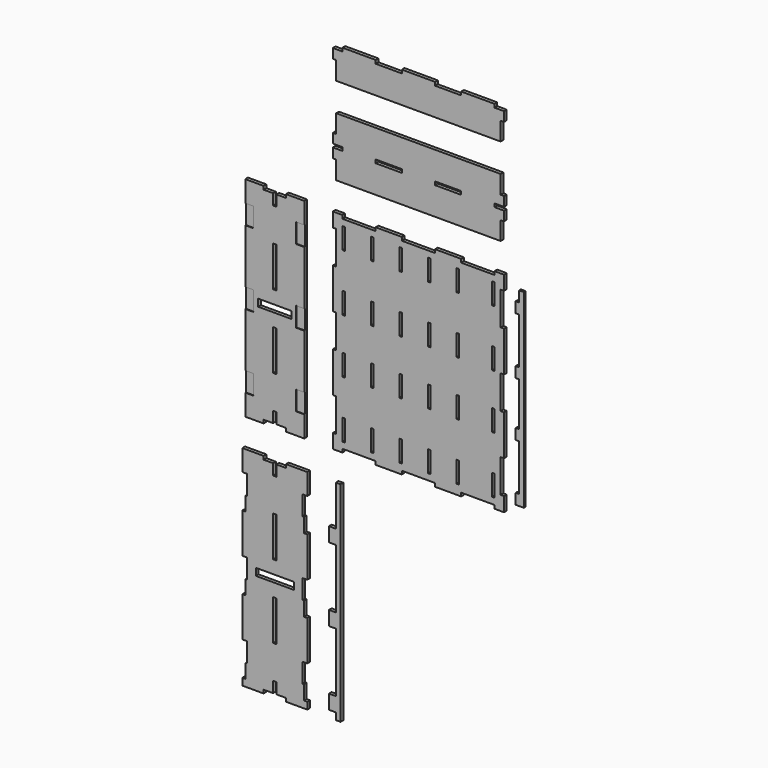
from build123d import *

# Parameters (mm, degrees)
F1_W     = 139.7
F1_H     = 18.034
F1_W_2   = 18.034
F1_H_2   = 50.8
F2_DEPTH = 18.034
F1_W_3   = 12.192
F1_H_3   = 113.5253
F1_H_4   = 215.9
F1_W_4   = 203.2
F1_H_5   = 38.1
F1_W_5   = 37.084
F1_H_6   = 76.2
F1_W_6   = 25.4
F1_H_7   = 217.17
F1_H_8   = 36.83
F1_W_7   = 177.8
F1_H_9   = 56.76265
F3_DEPTH = 12.192
F1_W_8   = 43.7134
F1_H_10  = 104.14
F4_DEPTH = 14.7574


# Not quite as in the source:
# - a variable given as a bare number and used for a length is read in inches; the dataset says mm whatever the document's units were
# - a feature names something its author has since deleted; it is built from what else it names


with BuildPart() as f2:
    # F1 (on Front) → F2 (new body)
    with BuildSketch(Plane.XZ):
        Polygon((439.166, 1026.668), (-439.166, 1026.668), (-439.166, 928.751), (-439.166, 877.951), (-406.4, 877.951), (-406.4, 859.917), (-439.166, 859.917), (-439.166, 809.117), (-439.166, 711.2), (439.166, 711.2), (439.166, 809.117), (439.166, 859.917), (406.4, 859.917), (406.4, 877.951), (439.166, 877.951), (439.166, 928.751), align=None)
        with Locations((-158.75, 868.934)):
            Rectangle(F1_W, F1_H, mode=Mode.SUBTRACT)
        with Locations((158.75, 868.934)):
            Rectangle(F1_W, F1_H, mode=Mode.SUBTRACT)
        with Locations((-448.183, 903.351)):
            Rectangle(F1_W_2, F1_H_2)
        with Locations((-448.183, 834.517)):
            Rectangle(F1_W_2, F1_H_2)
        with Locations((448.183, 903.351)):
            Rectangle(F1_W_2, F1_H_2)
        with Locations((448.183, 834.517)):
            Rectangle(F1_W_2, F1_H_2)
    extrude(amount=F2_DEPTH)


with BuildPart() as f2b:
    # F1 (on Front) → F2, piece 2 (new body)
    with BuildSketch(Plane.XZ):
        Polygon((-406.4, 558.8), (-457.2, 558.8), (-457.2, 482.6), (-439.166, 482.6), (-439.166, 304.8), (-457.2, 304.8), (-457.2, 88.9), (-439.166, 88.9), (-439.166, -88.9), (-457.2, -88.9), (-457.2, -304.8), (-439.166, -304.8), (-439.166, -482.6), (-457.2, -482.6), (-457.2, -558.8), (-406.4, -558.8), (-406.4, -540.766), (-228.6, -540.766), (-228.6, -558.8), (-88.9, -558.8), (-88.9, -540.766), (88.9, -540.766), (88.9, -558.8), (228.6, -558.8), (228.6, -540.766), (406.4, -540.766), (406.4, -558.8), (457.2, -558.8), (457.2, -482.6), (439.166, -482.6), (439.166, -304.8), (457.2, -304.8), (457.2, -88.9), (439.166, -88.9), (439.166, 88.9), (457.2, 88.9), (457.2, 304.8), (439.166, 304.8), (439.166, 482.6), (457.2, 482.6), (457.2, 558.8), (406.4, 558.8), (406.4, 540.766), (228.6, 540.766), (228.6, 558.8), (88.9, 558.8), (88.9, 540.766), (-88.9, 540.766), (-88.9, 558.8), (-228.6, 558.8), (-228.6, 540.766), (-406.4, 540.766), align=None)
        with Locations((-399.5293, -450.46265)):
            Rectangle(F1_W_3, F1_H_3, mode=Mode.SUBTRACT)
        with Locations((-247.1293, -450.46265)):
            Rectangle(F1_W_3, F1_H_3, mode=Mode.SUBTRACT)
        with Locations((-94.7293, -450.46265)):
            Rectangle(F1_W_3, F1_H_3, mode=Mode.SUBTRACT)
        with Locations((57.6707, -450.46265)):
            Rectangle(F1_W_3, F1_H_3, mode=Mode.SUBTRACT)
        with Locations((210.0707, -450.46265)):
            Rectangle(F1_W_3, F1_H_3, mode=Mode.SUBTRACT)
        with Locations((399.5293, -450.46265)):
            Rectangle(F1_W_3, F1_H_3, mode=Mode.SUBTRACT)
        with Locations((-399.5293, -145.66265)):
            Rectangle(F1_W_3, F1_H_3, mode=Mode.SUBTRACT)
        with Locations((-399.5293, 145.66265)):
            Rectangle(F1_W_3, F1_H_3, mode=Mode.SUBTRACT)
        with Locations((-247.1293, -145.66265)):
            Rectangle(F1_W_3, F1_H_3, mode=Mode.SUBTRACT)
        with Locations((-247.1293, 145.66265)):
            Rectangle(F1_W_3, F1_H_3, mode=Mode.SUBTRACT)
        with Locations((-399.5293, 450.46265)):
            Rectangle(F1_W_3, F1_H_3, mode=Mode.SUBTRACT)
        with Locations((-247.1293, 450.46265)):
            Rectangle(F1_W_3, F1_H_3, mode=Mode.SUBTRACT)
        with Locations((-94.7293, -145.66265)):
            Rectangle(F1_W_3, F1_H_3, mode=Mode.SUBTRACT)
        with Locations((-94.7293, 145.66265)):
            Rectangle(F1_W_3, F1_H_3, mode=Mode.SUBTRACT)
        with Locations((57.6707, -145.66265)):
            Rectangle(F1_W_3, F1_H_3, mode=Mode.SUBTRACT)
        with Locations((57.6707, 145.66265)):
            Rectangle(F1_W_3, F1_H_3, mode=Mode.SUBTRACT)
        with Locations((-94.7293, 450.46265)):
            Rectangle(F1_W_3, F1_H_3, mode=Mode.SUBTRACT)
        with Locations((57.6707, 450.46265)):
            Rectangle(F1_W_3, F1_H_3, mode=Mode.SUBTRACT)
        with Locations((210.0707, -145.66265)):
            Rectangle(F1_W_3, F1_H_3, mode=Mode.SUBTRACT)
        with Locations((210.0707, 145.66265)):
            Rectangle(F1_W_3, F1_H_3, mode=Mode.SUBTRACT)
        with Locations((399.5293, -145.66265)):
            Rectangle(F1_W_3, F1_H_3, mode=Mode.SUBTRACT)
        with Locations((399.5293, 145.66265)):
            Rectangle(F1_W_3, F1_H_3, mode=Mode.SUBTRACT)
        with Locations((210.0707, 450.46265)):
            Rectangle(F1_W_3, F1_H_3, mode=Mode.SUBTRACT)
        with Locations((399.5293, 450.46265)):
            Rectangle(F1_W_3, F1_H_3, mode=Mode.SUBTRACT)
    extrude(amount=F2_DEPTH)


with BuildPart() as f2c:
    # F1 (on Front) → F2, piece 3 (new body)
    with BuildSketch(Plane.XZ):
        Polygon((-439.166, 1276.985), (-439.166, 1179.068), (439.166, 1179.068), (439.166, 1276.985), (439.166, 1327.785), (406.4, 1327.785), (406.4, 1345.819), (228.6, 1345.819), (228.6, 1327.785), (88.9, 1327.785), (88.9, 1345.819), (-88.9, 1345.819), (-88.9, 1327.785), (-228.6, 1327.785), (-228.6, 1345.819), (-406.4, 1345.819), (-406.4, 1327.785), (-439.166, 1327.785), align=None)
        with Locations((448.183, 1302.385)):
            Rectangle(F1_W_2, F1_H_2)
        with Locations((-448.183, 1302.385)):
            Rectangle(F1_W_2, F1_H_2)
    extrude(amount=F2_DEPTH)


with BuildPart() as f2d:
    # F1 (on Front) → F2, piece 4 (new body)
    with BuildSketch(Plane.XZ):
        Polygon((-827.151, -711.2), (-940.943, -711.2), (-940.943, -824.23), (-915.543, -824.23), (-915.543, -928.37), (-922.909, -928.37), (-922.909, -1004.57), (-940.943, -1004.57), (-940.943, -1217.93), (-915.543, -1217.93), (-915.543, -1322.07), (-922.909, -1322.07), (-922.909, -1398.27), (-940.943, -1398.27), (-940.943, -1611.63), (-915.543, -1611.63), (-915.543, -1715.77), (-922.909, -1715.77), (-922.909, -1791.97), (-940.943, -1791.97), (-940.943, -1828.8), (-827.151, -1828.8), (-827.151, -1810.766), (-776.351, -1810.766), (-776.351, -1752.6), (-758.317, -1752.6), (-758.317, -1810.766), (-707.517, -1810.766), (-707.517, -1828.8), (-593.725, -1828.8), (-593.725, -1791.97), (-611.759, -1791.97), (-611.759, -1715.77), (-619.125, -1715.77), (-619.125, -1611.63), (-593.725, -1611.63), (-593.725, -1398.27), (-611.759, -1398.27), (-611.759, -1322.07), (-619.125, -1322.07), (-619.125, -1217.93), (-593.725, -1217.93), (-593.725, -1004.57), (-611.759, -1004.57), (-611.759, -928.37), (-619.125, -928.37), (-619.125, -824.23), (-593.725, -824.23), (-593.725, -711.2), (-707.517, -711.2), (-707.517, -729.234), (-758.317, -729.234), (-758.317, -787.4), (-776.351, -787.4), (-776.351, -729.234), (-827.151, -729.234), align=None)
        with Locations((-767.334, -1466.85)):
            Rectangle(F1_W_2, F1_H_4, mode=Mode.SUBTRACT)
        with Locations((-767.334, -1270)):
            Rectangle(F1_W_4, F1_H_5, mode=Mode.SUBTRACT)
        with Locations((-767.334, -1073.15)):
            Rectangle(F1_W_2, F1_H_4, mode=Mode.SUBTRACT)
    extrude(amount=F2_DEPTH)


with BuildPart() as f2e:
    # F1 (on Front) → F2, piece 5 (new body)
    with BuildSketch(Plane.XZ):
        with Locations((-459.867, -1360.17)):
            Rectangle(F1_W_5, F1_H_6)
        with Locations((-459.867, -1753.87)):
            Rectangle(F1_W_5, F1_H_6)
        Polygon((-415.925, -928.37), (-441.325, -928.37), (-441.325, -1004.57), (-441.325, -1322.07), (-441.325, -1398.27), (-441.325, -1715.77), (-441.325, -1791.97), (-415.925, -1791.97), align=None)
        with Locations((-459.867, -966.47)):
            Rectangle(F1_W_5, F1_H_6)
        with Locations((-428.625, -819.785)):
            Rectangle(F1_W_6, F1_H_7)
        with Locations((-428.625, -1810.385)):
            Rectangle(F1_W_6, F1_H_8)
    extrude(amount=F2_DEPTH)


with BuildPart() as f2f:
    # F1 (on Front) → F2, piece 6 (new body)
    with BuildSketch(Plane.XZ):
        Polygon((-707.517, -558.8), (-609.6, -558.8), (-609.6, -445.77), (-653.3134, -445.77), (-653.3134, -341.63), (-609.6, -341.63), (-609.6, -52.07), (-653.3134, -52.07), (-653.3134, 52.07), (-609.6, 52.07), (-609.6, 341.63), (-653.3134, 341.63), (-653.3134, 445.77), (-609.6, 445.77), (-609.6, 558.8), (-707.517, 558.8), (-707.517, 540.766), (-758.317, 540.766), (-758.317, 482.6), (-776.351, 482.6), (-776.351, 540.766), (-827.151, 540.766), (-827.151, 558.8), (-925.068, 558.8), (-925.068, 445.77), (-881.3546, 445.77), (-881.3546, 341.63), (-925.068, 341.63), (-925.068, 52.07), (-881.3546, 52.07), (-881.3546, -52.07), (-925.068, -52.07), (-925.068, -341.63), (-881.3546, -341.63), (-881.3546, -445.77), (-925.068, -445.77), (-925.068, -558.8), (-827.151, -558.8), (-827.151, -540.766), (-776.351, -540.766), (-776.351, -482.6), (-758.317, -482.6), (-758.317, -540.766), (-707.517, -540.766), align=None)
        with Locations((-767.334, -196.85)):
            Rectangle(F1_W_2, F1_H_4, mode=Mode.SUBTRACT)
        with Locations((-767.334, 0)):
            Rectangle(F1_W_7, F1_H_5, mode=Mode.SUBTRACT)
        with Locations((-767.334, 196.85)):
            Rectangle(F1_W_2, F1_H_4, mode=Mode.SUBTRACT)
    extrude(amount=F2_DEPTH)

    # F1 (on Front) → F4 (join)
    with BuildSketch(Plane.XZ):
        with Locations((-903.2113, 393.7)):
            Rectangle(F1_W_8, F1_H_10)
        with Locations((-631.4567, 393.7)):
            Rectangle(F1_W_8, F1_H_10)
        with Locations((-631.4567, 0)):
            Rectangle(F1_W_8, F1_H_10)
        with Locations((-903.2113, 0)):
            Rectangle(F1_W_8, F1_H_10)
        with Locations((-903.2113, -393.7)):
            Rectangle(F1_W_8, F1_H_10)
        with Locations((-631.4567, -393.7)):
            Rectangle(F1_W_8, F1_H_10)
    extrude(amount=F4_DEPTH)


with BuildPart() as f3:
    # F1 (on Front) → F3 (new body)
    with BuildSketch(Plane.XZ):
        Polygon((558.8, 507.2253), (533.4, 507.2253), (533.4, 450.46265), (533.4, 393.7), (533.4, 145.66265), (533.4, 88.9), (533.4, -145.66265), (533.4, -202.4253), (533.4, -450.46265), (533.4, -507.2253), (558.8, -507.2253), align=None)
        with Locations((524.383, 422.081325)):
            Rectangle(F1_W_2, F1_H_9)
        with Locations((524.383, 117.281325)):
            Rectangle(F1_W_2, F1_H_9)
        with Locations((524.383, -174.043975)):
            Rectangle(F1_W_2, F1_H_9)
        with Locations((524.383, -478.843975)):
            Rectangle(F1_W_2, F1_H_9)
    extrude(amount=F3_DEPTH)


solid = Compound([f2.part, f2b.part, f2c.part, f2d.part, f2e.part, f2f.part, f3.part])
